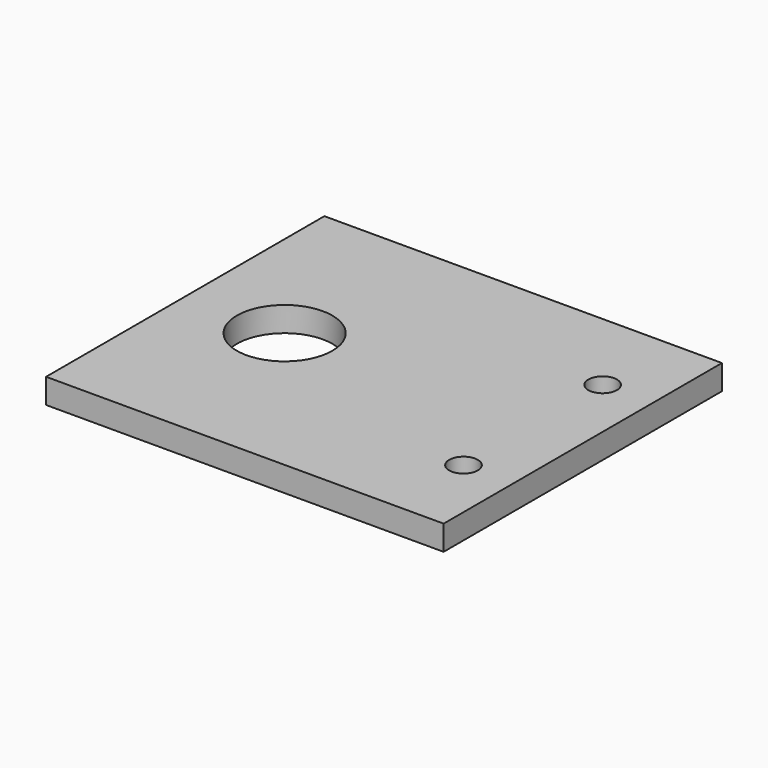
from build123d import *

# Parameters (mm, degrees)
F0_R     = 3.6643363337
F0_R_2   = 12.1990402392
F1_DEPTH = 6.35


# Not quite as in the source:
# - a feature names something its author has since deleted; it is built from what else it names


with BuildPart() as f1:
    # F0 (on Top) → F1 (new body)
    with BuildSketch(Plane.XY):
        Polygon((4.9436837435, 38.7340840895), (-45.8563162565, 38.7340840895), (-45.8563162565, -50.1659159105), (4.9436837435, -50.1659159105), (30.3436837435, -50.1659159105), (55.7436837435, -50.1659159105), (55.7436837435, -5.7159159105), (55.7436837435, 38.7340840895), (30.3436837435, 38.7340840895), align=None)
        with Locations((43.0436837435, -27.9409159105)):
            Circle(F0_R, mode=Mode.SUBTRACT)
        with Locations((-20.4563162565, -5.7159159105)):
            Circle(F0_R_2, mode=Mode.SUBTRACT)
        with Locations((43.0436837435, 16.5090840895)):
            Circle(F0_R, mode=Mode.SUBTRACT)
    extrude(amount=F1_DEPTH)


solid = f1.part
